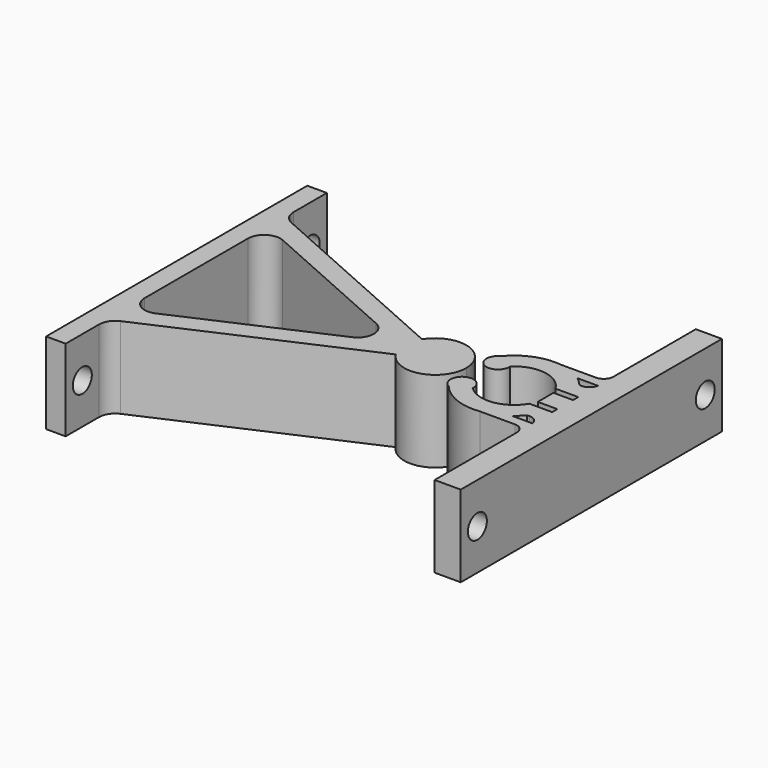
from build123d import *

# Parameters (mm, degrees)
F1_DEPTH      = 25
F2_R          = 5
F5_DEPTH      = 25
F3_R          = 3.6336150251
F6_DEPTH      = 6
F6_DEPTH_BACK = 121.001
F7_T1_DEPTH   = 25


# Not quite as in the source:
# - a fillet or chamfer that OpenCascade refuses, or shapes differently, is made with other operations: its cross-section is extruded or revolved along the edge and cut away or added


with BuildPart() as f1:
    # F0 (on Top) → F1 (new body)
    with BuildSketch(Plane.XY):
        Polygon((3, 34), (3, 50), (-3, 50), (-3, -50), (3, -50), (3, -34), (3, -27.4335767708), (3, 27.4335767708), align=None)
        with BuildLine():
            Line((68.1400732815, 5.0350114336), (3, 34))
            Line((3, 34), (3, 27.4335767708))
            Line((3, 27.4335767708), (64.6960437298, 0))
            Line((64.6960437298, 0), (3, -27.4335767708))
            Line((3, -27.4335767708), (3, -34))
            Line((3, -34), (68.1400732815, -5.0350114336))
            ThreePointArc((68.1400732815, -5.0350114336), (66.6960437298, 0), (68.1400732815, 5.0350114336))
        make_face()
        with BuildLine():
            ThreePointArc((85.6960437298, 0), (78.8150397914, 9.1318595932), (68.1400732815, 5.0350114336))
            ThreePointArc((68.1400732815, 5.0350114336), (66.6960437298, 0), (68.1400732815, -5.0350114336))
            ThreePointArc((68.1400732815, -5.0350114336), (78.8150397914, -9.1318595932), (85.6960437298, 0))
        make_face()
    extrude(amount=F1_DEPTH)

    # F2
    f2_edges = [f1.edges().sort_by_distance(p)[0] for p in [
        (64.696044, 0, 12.5),
        (3, 27.433577, 12.5),
        (3, -27.433577, 12.5),
        (3, 34, 12.5),
        (3, -34, 12.5),
    ]]
    fillet(f2_edges, radius=F2_R)


with BuildPart() as f5:
    # F4 (on Top) → F5 (new body)
    with BuildSketch(Plane.XY):
        Polygon((124, -50), (124, 50), (116, 50), (116, 15.5), (116, 12.5), (116, 10), (116, 5), (116, 3), (116, -3), (116, -5), (116, -10), (116, -12.5), (116, -15.5), (116, -50), align=None)
        with BuildLine():
            Line((116, 12.5), (116, 15.5))
            Line((116, 15.5), (102.3548491623, 15.5))
            ThreePointArc((102.3548491623, 15.5), (106.233407666, 14.476718987), (109.7238090964, 12.5))
            Line((109.7238090964, 12.5), (116, 12.5))
        make_face()
        with BuildLine():
            ThreePointArc((109.7238090964, 12.5), (106.233407666, 14.476718987), (102.3548491623, 15.5))
            ThreePointArc((102.3548491623, 15.5), (94.6343391262, 14.551940549), (88.326809564, 10))
            ThreePointArc((88.326809564, 10), (91.6045970412, 9.9418299371), (93.3963954262, 7.1965188345))
            ThreePointArc((93.3963954262, 7.1965188345), (101.7337018999, 9.9023677393), (109, 5))
            Line((109, 5), (115.1488864135, 5))
            Line((115.1488864135, 5), (116, 5))
            Line((116, 5), (116, 10))
            Line((116, 10), (112.3526823604, 10))
            ThreePointArc((112.3526823604, 10), (111.1110224533, 11.3265283145), (109.7238090964, 12.5))
        make_face()
        with BuildLine():
            Line((102.3548491623, -15.5), (116, -15.5))
            Line((116, -15.5), (116, -12.5))
            Line((116, -12.5), (109.7238090964, -12.5))
            ThreePointArc((109.7238090964, -12.5), (106.233407666, -14.476718987), (102.3548491623, -15.5))
        make_face()
        with BuildLine():
            ThreePointArc((93.3963954262, 7.1965188345), (91.6045970412, 9.9418299371), (88.326809564, 10))
            ThreePointArc((88.326809564, 10), (88.0797216709, 3.8961721588), (93.4108312054, 6.8789624418))
            ThreePointArc((93.4108312054, 6.8789624418), (93.407220398, 7.0379046123), (93.3963954262, 7.1965188345))
        make_face()
        with BuildLine():
            ThreePointArc((88.326809564, -10), (94.6343391262, -14.551940549), (102.3548491623, -15.5))
            ThreePointArc((102.3548491623, -15.5), (106.233407666, -14.476718987), (109.7238090964, -12.5))
            ThreePointArc((109.7238090964, -12.5), (111.1110224533, -11.3265283145), (112.3526823604, -10))
            Line((112.3526823604, -10), (116, -10))
            Line((116, -10), (116, -5))
            Line((116, -5), (115.1488864135, -5))
            Line((115.1488864135, -5), (109, -5))
            ThreePointArc((109, -5), (101.7337018999, -9.9023677393), (93.3963954262, -7.1965188345))
            ThreePointArc((93.3963954262, -7.1965188345), (91.6045970412, -9.9418299371), (88.326809564, -10))
        make_face()
        with BuildLine():
            ThreePointArc((93.4108312054, -6.8789624418), (88.0797216709, -3.8961721588), (88.326809564, -10))
            ThreePointArc((88.326809564, -10), (91.6045970412, -9.9418299371), (93.3963954262, -7.1965188345))
            ThreePointArc((93.3963954262, -7.1965188345), (93.407220398, -7.0379046123), (93.4108312054, -6.8789624418))
        make_face()
        Polygon((116, -3), (116, 3), (110, 3), (110, 0), (110, -3), align=None)
    extrude(amount=F5_DEPTH)


with BuildPart() as f6_tool:
    # F3 (on face) → F6 (new body, two sides)
    with BuildSketch(Plane.YZ.offset(3)) as f6_sk:
        with Locations((-43.6243672171, 12.5)):
            Circle(F3_R)
        with Locations((43.6243672171, 12.5)):
            Circle(F3_R)
    extrude(amount=-F6_DEPTH)
    extrude(f6_sk.sketch, amount=F6_DEPTH_BACK)


with BuildPart() as f1_1:
    add(f1.part)

    # F6: cut by f6_tool
    add(f6_tool.part, mode=Mode.SUBTRACT)


with BuildPart() as f5_1:
    add(f5.part)

    # F6: cut by f6_tool
    add(f6_tool.part, mode=Mode.SUBTRACT)

    # F7: fillet of radius 3 on 4 edges, made by hand

    # F7_s2 → F7_t1 (join)
    with BuildSketch(Plane.XY):
        with BuildLine():
            ThreePointArc((116, 12.5), (114.9784517816, 10.7087121525), (113.0419601084, 10))
            Line((113.0419601084, 10), (116, 10))
            Line((116, 10), (116, 12.5))
        make_face()
        with BuildLine():
            ThreePointArc((116, -12.5), (114.9784517816, -10.7087121525), (113.0419601085, -10))
            Line((113.0419601085, -10), (116, -10))
            Line((116, -10), (116, -12.5))
        make_face()
        with BuildLine():
            ThreePointArc((116, -18.5), (115.1213203436, -16.3786796564), (113, -15.5))
            Line((113, -15.5), (116, -15.5))
            Line((116, -15.5), (116, -18.5))
        make_face()
        with BuildLine():
            ThreePointArc((116, 18.5), (115.1213203436, 16.3786796564), (113, 15.5))
            Line((113, 15.5), (116, 15.5))
            Line((116, 15.5), (116, 18.5))
        make_face()
    extrude(amount=F7_T1_DEPTH)


solid = Compound([f1_1.part, f5_1.part])
